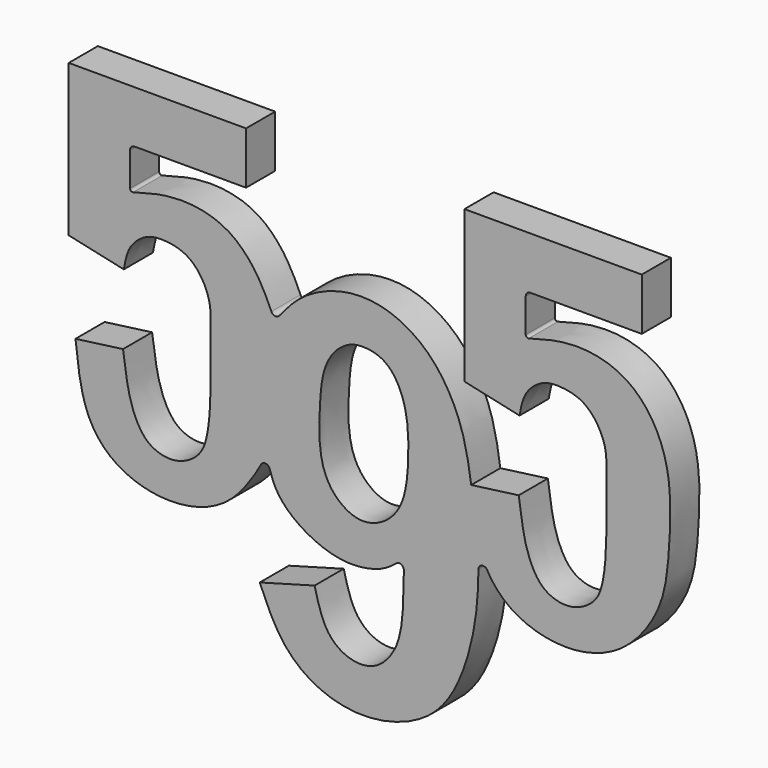
from build123d import *

# Parameters (mm, degrees)
F1_DEPTH = 3


with BuildPart() as f1:
    # F0 (on Front) → F1 (new body)
    with BuildSketch(Plane.XZ):
        with BuildLine():
            Line((-9.5692276955, 19.0295055509), (-24.1804867983, 19.0295055509))
            Line((-24.1804867983, 19.0295055509), (-24.1804867983, 6.5188668668))
            Line((-24.1804867983, 6.5188668668), (-19.641533494, 5.5243223906))
            add(Edge.make_bspline(
                [(-19.7093635798, -0.2800785005), (-19.5570157915, -1.4128068863), (-19.2832323204, -3.4484279333), (-18.5109109074, -5.4535206804), (-17.4051281218, -6.7542628508), (-15.3991816922, -7.2105429933), (-13.5454389459, -6.2089714944), (-12.6915145355, -4.6565826928), (-12.4086880358, -0.8100851133), (-12.5420416876, 3.029626915), (-12.3568219976, 5.7747033617), (-14.0206086131, 8.3373482447), (-16.2066326759, 8.7783260416), (-17.7914404465, 8.6742253566), (-19.3296180044, 7.3709317022), (-19.5261044193, 6.1267789414), (-19.641533494, 5.5243223906)],
                knots=[0, 0, 0, 0, 0.0850530681, 0.1531982013, 0.2128134932, 0.2778382163, 0.3433024412, 0.4040377865, 0.4960108059, 0.5899390151, 0.6674603836, 0.7458264942, 0.8140016254, 0.8723646786, 0.9361011897, 1, 1, 1, 1], degree=3))
            Line((-19.7093635798, -0.2800785005), (-23.6246287823, -0.8048042655))
            add(Edge.make_bspline(
                [(-23.6246287823, -0.8048042655), (-23.4238768593, -2.6360165944), (-23.0505161222, -6.0417263616), (-20.3186102891, -9.2347391659), (-15.6652683934, -10.4746071304), (-10.9657366753, -9.1109706503), (-8.8996831286, -5.9644979669), (-8.4359519706, -5.1438258987), (-8.3332477687, -4.9554002855)],
                knots=[0, 0, 0, 0, 0.1973470203, 0.3670282598, 0.5513187137, 0.7396844469, 0.9084969392, 0.9665234371, 0.9665234371, 0.9665234371, 0.9665234371], degree=3))
            ThreePointArc((-8.3332477687, -4.9554002855), (-7.954646037, -4.7561731868), (-7.6247713503, -5.0285945502))
            add(Edge.make_bspline(
                [(-7.6247713503, -5.0285945502), (-7.4951246028, -5.4581028515), (-7.1182427223, -6.5417591982), (-5.5143339169, -8.3435497571), (-1.8620178866, -10.0886878273), (1.4142697444, -9.5568731886), (2.461744348, -8.7898311991), (2.804982612, -8.5018005366)],
                knots=[0.0376498734, 0.0376498734, 0.0376498734, 0.0376498734, 0.1637941515, 0.3576495972, 0.6037857722, 0.8301707333, 0.9551635836, 0.9551635836, 0.9551635836, 0.9551635836], degree=3))
            ThreePointArc((2.804982612, -8.5018005366), (3.2178473715, -8.4483976929), (3.4391110044, -8.801032884))
            add(Edge.make_bspline(
                [(3.4391110044, -8.801032884), (3.4292294296, -9.8788771881), (3.3907020801, -12.0466383407), (2.98547267, -14.7224859441), (1.1638632401, -16.8474068921), (-1.2378962082, -16.8165054966), (-3.15517022, -15.3270751162), (-3.6508764536, -13.3639063953), (-3.91946733, -12.3001933098)],
                knots=[0.0310308646, 0.0310308646, 0.0310308646, 0.0310308646, 0.1949538702, 0.364973689, 0.5249423704, 0.6722147355, 0.8223945444, 1, 1, 1, 1], degree=3))
            Line((-3.91946733, -12.3001933098), (-8.4416717291, -13.5454395786))
            add(Edge.make_bspline(
                [(-8.4416717291, -13.5454395786), (-7.9438695099, -14.71578707), (-6.9579408758, -17.0337339557), (-4.2409263056, -19.6699254166), (0.459261844, -20.936928095), (5.9462638445, -19.1007566385), (8.4575100908, -14.8113966737), (9.4779663102, -10.267236628), (9.5666941787, -7.7613995922), (9.583580391, -6.731421425)],
                knots=[0, 0, 0, 0, 0.131573279, 0.2605891623, 0.4072468832, 0.5651074981, 0.7133867816, 0.8642572868, 0.9719474004, 0.9719474004, 0.9719474004, 0.9719474004], degree=3))
            ThreePointArc((9.583580391, -6.731421425), (9.8768736928, -6.3630255441), (10.3080651221, -6.5522620029))
            add(Edge.make_bspline(
                [(10.3080651221, -6.5522620029), (10.1985750854, -6.3524360688), (9.4191824802, -4.7382862047), (9.1880568861, -2.6361142764), (8.9867115021, -0.8048042655)],
                knots=[0.8907000755, 0.8907000755, 0.8907000755, 0.8907000755, 0.9047832181, 1, 1, 1, 1], degree=3))
            add(Edge.make_bspline(
                [(-6.8268028651, 6.3355319618), (-6.3239368021, 6.9578108483), (-5.1657820011, 8.33523566), (-2.1396728387, 9.9326729538), (1.8950429815, 10.0853631714), (6.0194775368, 7.6605840045), (8.3949703412, 3.199174132), (8.7962173797, 0.4841619269), (8.9867115021, -0.8048042655)],
                knots=[0.0134429235, 0.0134429235, 0.0134429235, 0.0134429235, 0.1392843233, 0.2952512735, 0.4619051388, 0.6427907875, 0.8304130649, 1, 1, 1, 1], degree=3))
            ThreePointArc((-6.8268028651, 6.3355319618), (-7.1773938737, 6.1954394373), (-7.479812433, 6.4214548917))
            add(Edge.make_bspline(
                [(-18.8772828528, 11.3704401816), (-18.0907039553, 11.5942528357), (-16.428571119, 12.048986212), (-13.7637590064, 12.1663926481), (-10.7783023467, 11.2878918717), (-8.608008816, 8.883739189), (-7.8235892044, 7.195407339), (-7.479812433, 6.4214548917)],
                knots=[0.0187889452, 0.0187889452, 0.0187889452, 0.0187889452, 0.1928215696, 0.3859968189, 0.5892635727, 0.8004585236, 0.9781550685, 0.9781550685, 0.9781550685, 0.9781550685], degree=3))
            ThreePointArc((-18.8772828528, 11.3704401816), (-19.052543922, 11.4032002875), (-19.1320180893, 11.5628045595))
            Line((-19.1320180893, 11.5628045595), (-19.1320180893, 14.3393719836))
            ThreePointArc((-19.1320180893, 14.3393719836), (-19.0189579715, 14.6123232533), (-18.7460067018, 14.7253833711))
            Line((-18.7460067018, 14.7253833711), (-9.5692276955, 14.7253833711))
            Line((-9.5692276955, 14.7253833711), (-9.5692276955, 19.0295055509))
        make_face()
        with BuildLine():
            add(Edge.make_bspline(
                [(-3.4354478121, 1.6201604158), (-3.5268113996, 0.5204862984), (-3.661245232, -2.1514122715), (-2.8038980937, -5.0376153478), (-0.0082786462, -6.9479730958), (3.4625349906, -4.9889346896), (3.899180856, -0.526341138), (3.7411706941, 3.4063941992), (2.0399404478, 6.2494758513), (-0.4779286797, 6.4088353336), (-1.415072846, 5.9485227508), (-2.3566320655, 5.2360821356), (-3.2138401141, 3.6852138136), (-3.3662258173, 2.4533329967), (-3.4354478121, 1.6201604158)],
                knots=[0, 0, 0, 0, 0.1002894958, 0.1897756028, 0.2774641613, 0.3709145582, 0.478467765, 0.5828122225, 0.6726179006, 0.7498518805, 0.8019038103, 0.8568491044, 0.9240152544, 1, 1, 1, 1], degree=3))
        make_face(mode=Mode.SUBTRACT)
        with BuildLine():
            Line((12.9019767046, -0.2800785005), (8.9867115021, -0.8048042655))
            add(Edge.make_bspline(
                [(10.3080651221, -6.5522620029), (10.1985750854, -6.3524360688), (9.4191824802, -4.7382862047), (9.1880568861, -2.6361142764), (8.9867115021, -0.8048042655)],
                knots=[0.8907000755, 0.8907000755, 0.8907000755, 0.8907000755, 0.9047832181, 1, 1, 1, 1], degree=3))
            add(Edge.make_bspline(
                [(13.7339183255, 11.370197343), (14.5206329081, 11.5934338311), (16.1829432155, 12.0472832886), (18.8464510581, 12.1747073507), (21.8375982381, 11.2543430537), (24.2004389296, 8.7818679608), (25.5755735256, 4.8713271716), (25.3064350862, -0.5737911857), (24.8312041176, -4.7094018545), (21.749976272, -9.0376680335), (16.9706732988, -10.4786564529), (12.5389209811, -9.3007692118), (10.8350653675, -7.5140693006), (10.3080651221, -6.5522620029)],
                knots=[0.006673314, 0.006673314, 0.006673314, 0.006673314, 0.0685294658, 0.1371846306, 0.2094263518, 0.2844857821, 0.3685608886, 0.4653028232, 0.5506041076, 0.6431140813, 0.7339975358, 0.8229147331, 0.8907000755, 0.8907000755, 0.8907000755, 0.8907000755], degree=3))
            ThreePointArc((13.7339183255, 11.370197343), (13.5587386682, 11.40304056), (13.4793221951, 11.5626012477))
            Line((13.4793221951, 11.5626012477), (13.4793221951, 14.3393719836))
            ThreePointArc((13.4793221951, 14.3393719836), (13.5923823128, 14.6123232533), (13.8653335825, 14.7253833711))
            Line((13.8653335825, 14.7253833711), (23.0421125889, 14.7253833711))
            Line((23.0421125889, 14.7253833711), (23.0421125889, 19.0295055509))
            Line((23.0421125889, 19.0295055509), (8.4308534861, 19.0295055509))
            Line((8.4308534861, 19.0295055509), (8.4308534861, 6.5188668668))
            Line((8.4308534861, 6.5188668668), (12.9698067904, 5.5243223906))
            add(Edge.make_bspline(
                [(12.9019767046, -0.2800785005), (13.0543244929, -1.4128068863), (13.328107964, -3.4484279333), (14.1004293769, -5.4535206804), (15.2062121625, -6.7542628508), (17.2121585921, -7.2105429933), (19.0659013385, -6.2089714944), (19.9198257488, -4.6565826928), (20.2026522486, -0.8100851133), (20.0692985967, 3.029626915), (20.2545182868, 5.7747033617), (18.5907316712, 8.3373482447), (16.4047076085, 8.7783260416), (14.8198998378, 8.6742253566), (13.28172228, 7.3709317022), (13.085235865, 6.1267789414), (12.9698067904, 5.5243223906)],
                knots=[0, 0, 0, 0, 0.0850530681, 0.1531982013, 0.2128134932, 0.2778382163, 0.3433024412, 0.4040377865, 0.4960108059, 0.5899390151, 0.6674603836, 0.7458264942, 0.8140016254, 0.8723646786, 0.9361011897, 1, 1, 1, 1], degree=3))
        make_face()
    extrude(amount=F1_DEPTH)


solid = f1.part
